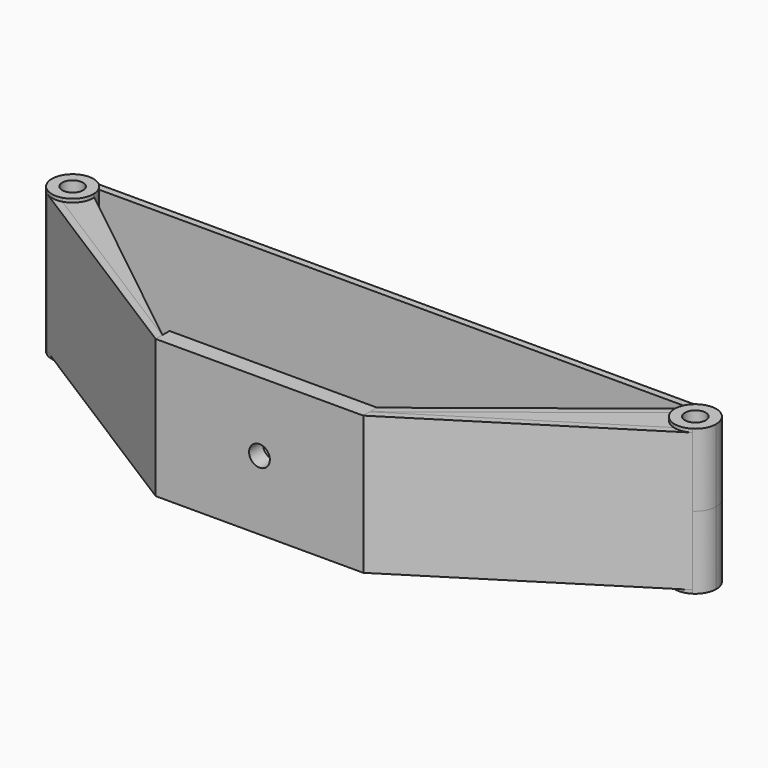
from build123d import *

# Parameters (mm, degrees)
F1_START      = -15
F0_R          = 3
F1_DEPTH      = 5
F2_DEPTH      = 20
F3_START      = -17
F3_DEPTH      = 3
F4_START      = 15
F4_DEPTH      = 5
F5_DEPTH      = 21
F5_DEPTH_BACK = 21
F6_R          = 3
F7_DEPTH      = 5
F8_DEPTH      = 20
F8_DEPTH_BACK = 20
F9_DEPTH      = 20
F9_DEPTH_BACK = 20


with BuildPart() as f1:
    # F0 (on Top) → F1 (new body)
    with BuildSketch(Plane.XY.offset(F1_START)):
        with BuildLine():
            Line((-93.2044615088, 39.927384655), (-30, 0))
            Line((-30, 0), (-30, 2.3656435948))
            Line((-30, 2.3656435948), (-88.3554034274, 39.2297918483))
            ThreePointArc((-88.3554034274, 39.2297918483), (-90.8543732122, 39.0611409838), (-93.2044615088, 39.927384655))
        make_face()
        with BuildLine():
            Line((-88.3554034274, 39.2297918483), (-30, 2.3656435948))
            Line((-30, 2.3656435948), (-30, 2.4457583538))
            Line((-30, 2.4457583538), (-84.0102370798, 45.3503429172))
            ThreePointArc((-84.0102370798, 45.3503429172), (-84.002559816, 45.175246225), (-84, 45))
            ThreePointArc((-84, 45), (-85.2110763508, 41.3852786716), (-88.3554034274, 39.2297918483))
        make_face()
        with BuildLine():
            ThreePointArc((-90, 51), (-95.7634925206, 46.6679790061), (-93.2044615088, 39.927384655))
            ThreePointArc((-93.2044615088, 39.927384655), (-90.8543732122, 39.0611409838), (-88.3554034274, 39.2297918483))
            ThreePointArc((-88.3554034274, 39.2297918483), (-85.2110763508, 41.3852786716), (-84, 45))
            ThreePointArc((-84, 45), (-84.002559816, 45.175246225), (-84.0102370798, 45.3503429172))
            ThreePointArc((-84.0102370798, 45.3503429172), (-84.4598888798, 47.3037293191), (-85.527864045, 49))
            ThreePointArc((-85.527864045, 49), (-85.8830871702, 49.3647484179), (-86.2679549126, 49.698067631))
            ThreePointArc((-86.2679549126, 49.698067631), (-88.0236910396, 50.6651745686), (-90, 51))
        make_face()
        with Locations((-90, 45)):
            Circle(F0_R, mode=Mode.SUBTRACT)
    extrude(amount=-F1_DEPTH)


with BuildPart() as f1b:
    # F0 (on Top) → F1, piece 2 (new body)
    with BuildSketch(Plane.XY.offset(F1_START)):
        with BuildLine():
            Line((30, 2.3656435948), (30, 0))
            Line((30, 0), (93.2044615088, 39.927384655))
            ThreePointArc((93.2044615088, 39.927384655), (90.8543732122, 39.0611409838), (88.3554034274, 39.2297918483))
            Line((88.3554034274, 39.2297918483), (30, 2.3656435948))
        make_face()
        with BuildLine():
            Line((30, 2.4538071327), (30, 2.3656435948))
            Line((30, 2.3656435948), (88.3554034274, 39.2297918483))
            ThreePointArc((88.3554034274, 39.2297918483), (85.2110763508, 41.3852786716), (84, 45))
            Line((84, 45), (30, 2.4538071327))
        make_face()
        with BuildLine():
            ThreePointArc((88.3554034274, 39.2297918483), (90.8543732122, 39.0611409838), (93.2044615088, 39.927384655))
            ThreePointArc((93.2044615088, 39.927384655), (95.2548439107, 42.1040346215), (96, 45))
            ThreePointArc((96, 45), (94.2426406871, 49.2426406871), (90, 51))
            ThreePointArc((90, 51), (87.5505102572, 50.4772255751), (85.527864045, 49))
            ThreePointArc((85.527864045, 49), (85.2652230991, 48.6853612711), (85.0246748585, 48.3535264627))
            ThreePointArc((85.0246748585, 48.3535264627), (84.261883983, 46.7532896439), (84, 45))
            ThreePointArc((84, 45), (85.2110763508, 41.3852786716), (88.3554034274, 39.2297918483))
        make_face()
        with Locations((90, 45)):
            Circle(F0_R, mode=Mode.SUBTRACT)
        with BuildLine():
            Line((30, 5), (30, 2.4538071327))
            Line((30, 2.4538071327), (84, 45))
            ThreePointArc((84, 45), (84.261883983, 46.7532896439), (85.0246748585, 48.3535264627))
            Line((85.0246748585, 48.3535264627), (30, 5))
        make_face()
    extrude(amount=-F1_DEPTH)


with BuildPart() as f2:
    # F0 (on Top) → F2 (new body, symmetric)
    with BuildSketch(Plane.XY):
        Polygon((-30, 2.3656435948), (-30, 0), (30, 0), (30, 2.3656435948), (30, 2.4538071327), (30, 5), (-30, 5), (-30, 2.4457583538), align=None)
    extrude(amount=F2_DEPTH, both=True)

    # F0 (on Top) → F4 (join)
    with BuildSketch(Plane.XY.offset(F4_START)):
        with BuildLine():
            Line((-93.2044615088, 39.927384655), (-30, 0))
            Line((-30, 0), (-30, 2.3656435948))
            Line((-30, 2.3656435948), (-88.3554034274, 39.2297918483))
            ThreePointArc((-88.3554034274, 39.2297918483), (-90.8543732122, 39.0611409838), (-93.2044615088, 39.927384655))
        make_face()
        with BuildLine():
            Line((30, 2.3656435948), (30, 0))
            Line((30, 0), (93.2044615088, 39.927384655))
            ThreePointArc((93.2044615088, 39.927384655), (90.8543732122, 39.0611409838), (88.3554034274, 39.2297918483))
            Line((88.3554034274, 39.2297918483), (30, 2.3656435948))
        make_face()
        with BuildLine():
            Line((-88.3554034274, 39.2297918483), (-30, 2.3656435948))
            Line((-30, 2.3656435948), (-30, 2.4457583538))
            Line((-30, 2.4457583538), (-84.0102370798, 45.3503429172))
            ThreePointArc((-84.0102370798, 45.3503429172), (-84.002559816, 45.175246225), (-84, 45))
            ThreePointArc((-84, 45), (-85.2110763508, 41.3852786716), (-88.3554034274, 39.2297918483))
        make_face()
        with BuildLine():
            Line((30, 2.4538071327), (30, 2.3656435948))
            Line((30, 2.3656435948), (88.3554034274, 39.2297918483))
            ThreePointArc((88.3554034274, 39.2297918483), (85.2110763508, 41.3852786716), (84, 45))
            Line((84, 45), (30, 2.4538071327))
        make_face()
        with BuildLine():
            Line((30, 5), (30, 2.4538071327))
            Line((30, 2.4538071327), (84, 45))
            ThreePointArc((84, 45), (84.261883983, 46.7532896439), (85.0246748585, 48.3535264627))
            Line((85.0246748585, 48.3535264627), (30, 5))
        make_face()
    extrude(amount=F4_DEPTH)

    # F6 (on Front) → F7 (cut)
    with BuildSketch(Plane.XZ):
        Circle(F6_R)
    extrude(amount=-F7_DEPTH, mode=Mode.SUBTRACT)


with BuildPart() as f3:
    # F0 (on Top) → F3 (new body)
    with BuildSketch(Plane.XY.offset(F3_START)):
        with BuildLine():
            Line((-85.3891957163, 49), (-30, 5))
            Line((-30, 5), (30, 5))
            Line((30, 5), (85.0246748585, 48.3535264627))
            ThreePointArc((85.0246748585, 48.3535264627), (85.2652230991, 48.6853612711), (85.527864045, 49))
            Line((85.527864045, 49), (-85.3891957163, 49))
        make_face()
    extrude(amount=-F3_DEPTH)


with BuildPart() as f5:
    # F0 (on Top) → F5 (new body, two sides)
    with BuildSketch(Plane.XY) as f5_sk:
        with BuildLine():
            ThreePointArc((-90, 51), (-95.7634925206, 46.6679790061), (-93.2044615088, 39.927384655))
            ThreePointArc((-93.2044615088, 39.927384655), (-90.8543732122, 39.0611409838), (-88.3554034274, 39.2297918483))
            ThreePointArc((-88.3554034274, 39.2297918483), (-85.2110763508, 41.3852786716), (-84, 45))
            ThreePointArc((-84, 45), (-84.002559816, 45.175246225), (-84.0102370798, 45.3503429172))
            ThreePointArc((-84.0102370798, 45.3503429172), (-84.4598888798, 47.3037293191), (-85.527864045, 49))
            ThreePointArc((-85.527864045, 49), (-85.8830871702, 49.3647484179), (-86.2679549126, 49.698067631))
            ThreePointArc((-86.2679549126, 49.698067631), (-88.0236910396, 50.6651745686), (-90, 51))
        make_face()
        with Locations((-90, 45)):
            Circle(F0_R, mode=Mode.SUBTRACT)
    extrude(amount=F5_DEPTH)
    extrude(f5_sk.sketch, amount=-F5_DEPTH_BACK)


with BuildPart() as f5b:
    # F0 (on Top) → F5, piece 2 (new body, two sides)
    with BuildSketch(Plane.XY) as f5_2_sk:
        with BuildLine():
            ThreePointArc((88.3554034274, 39.2297918483), (90.8543732122, 39.0611409838), (93.2044615088, 39.927384655))
            ThreePointArc((93.2044615088, 39.927384655), (95.2548439107, 42.1040346215), (96, 45))
            ThreePointArc((96, 45), (94.2426406871, 49.2426406871), (90, 51))
            ThreePointArc((90, 51), (87.5505102572, 50.4772255751), (85.527864045, 49))
            ThreePointArc((85.527864045, 49), (85.2652230991, 48.6853612711), (85.0246748585, 48.3535264627))
            ThreePointArc((85.0246748585, 48.3535264627), (84.261883983, 46.7532896439), (84, 45))
            ThreePointArc((84, 45), (85.2110763508, 41.3852786716), (88.3554034274, 39.2297918483))
        make_face()
        with Locations((90, 45)):
            Circle(F0_R, mode=Mode.SUBTRACT)
    extrude(amount=F5_DEPTH)
    extrude(f5_2_sk.sketch, amount=-F5_DEPTH_BACK)


with BuildPart() as f8:
    # F0 (on Top) → F8 (new body, two sides)
    with BuildSketch(Plane.XY) as f8_sk:
        with BuildLine():
            Line((-93.2044615088, 39.927384655), (-30, 0))
            Line((-30, 0), (-30, 2.3656435948))
            Line((-30, 2.3656435948), (-88.3554034274, 39.2297918483))
            ThreePointArc((-88.3554034274, 39.2297918483), (-90.8543732122, 39.0611409838), (-93.2044615088, 39.927384655))
        make_face()
    extrude(amount=F8_DEPTH)
    extrude(f8_sk.sketch, amount=-F8_DEPTH_BACK)


with BuildPart() as f8b:
    # F0 (on Top) → F8, piece 2 (new body, two sides)
    with BuildSketch(Plane.XY) as f8_2_sk:
        with BuildLine():
            Line((30, 2.3656435948), (30, 0))
            Line((30, 0), (93.2044615088, 39.927384655))
            ThreePointArc((93.2044615088, 39.927384655), (90.8543732122, 39.0611409838), (88.3554034274, 39.2297918483))
            Line((88.3554034274, 39.2297918483), (30, 2.3656435948))
        make_face()
    extrude(amount=F8_DEPTH)
    extrude(f8_2_sk.sketch, amount=-F8_DEPTH_BACK)


with BuildPart() as f8c:
    # F0 (on Top) → F8, piece 3 (new body, two sides)
    with BuildSketch(Plane.XY) as f8_3_sk:
        with BuildLine():
            Line((30, 5), (30, 2.4538071327))
            Line((30, 2.4538071327), (84, 45))
            ThreePointArc((84, 45), (84.261883983, 46.7532896439), (85.0246748585, 48.3535264627))
            Line((85.0246748585, 48.3535264627), (30, 5))
        make_face()
    extrude(amount=F8_DEPTH)
    extrude(f8_3_sk.sketch, amount=-F8_DEPTH_BACK)


with BuildPart() as f8d:
    # F0 (on Top) → F8, piece 4 (new body, two sides)
    with BuildSketch(Plane.XY) as f8_4_sk:
        with BuildLine():
            Line((-85.3891957163, 49), (-86.2679549126, 49.698067631))
            ThreePointArc((-86.2679549126, 49.698067631), (-85.8830871702, 49.3647484179), (-85.527864045, 49))
            Line((-85.527864045, 49), (-85.3891957163, 49))
        make_face()
    extrude(amount=F8_DEPTH)
    extrude(f8_4_sk.sketch, amount=-F8_DEPTH_BACK)


with BuildPart() as f9:
    # F0 (on Top) → F9 (new body, two sides)
    with BuildSketch(Plane.XY) as f9_sk:
        with BuildLine():
            Line((90, 51), (-90, 51))
            ThreePointArc((-90, 51), (-88.0236910396, 50.6651745686), (-86.2679549126, 49.698067631))
            Line((-86.2679549126, 49.698067631), (-85.3891957163, 49))
            Line((-85.3891957163, 49), (85.527864045, 49))
            ThreePointArc((85.527864045, 49), (87.5505102572, 50.4772255751), (90, 51))
        make_face()
    extrude(amount=F9_DEPTH)
    extrude(f9_sk.sketch, amount=-F9_DEPTH_BACK)


solid = Compound([f1.part, f1b.part, f2.part, f3.part, f5.part, f5b.part, f8.part, f8b.part, f8c.part, f8d.part, f9.part])
